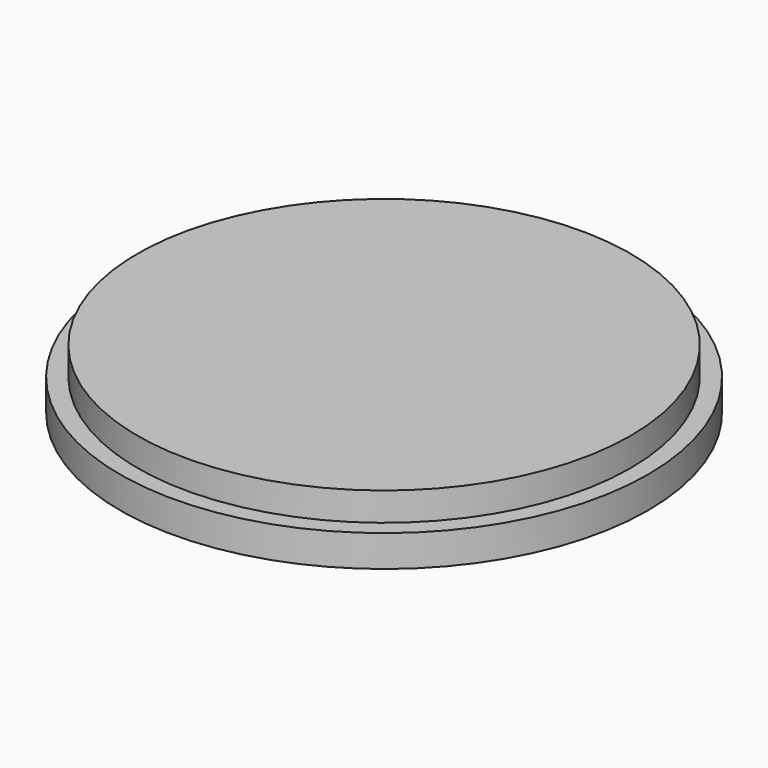
from build123d import *

# Parameters (mm, degrees)
F0_R     = 78
F1_DEPTH = 19
F0_R_2   = 83.5
F2_DEPTH = 10


# Not quite as in the source:
# - a feature of the source that left no trace in its solid (it failed there, or was rolled back) is left out


with BuildPart() as f1:
    # F0 (on Top) → F1 (new body)
    with BuildSketch(Plane.XY):
        Circle(F0_R)
    extrude(amount=F1_DEPTH)

    # F0 (on Top) → F2 (join)
    with BuildSketch(Plane.XY):
        Circle(F0_R_2)
        Circle(F0_R, mode=Mode.SUBTRACT)
    extrude(amount=F2_DEPTH)


solid = f1.part
